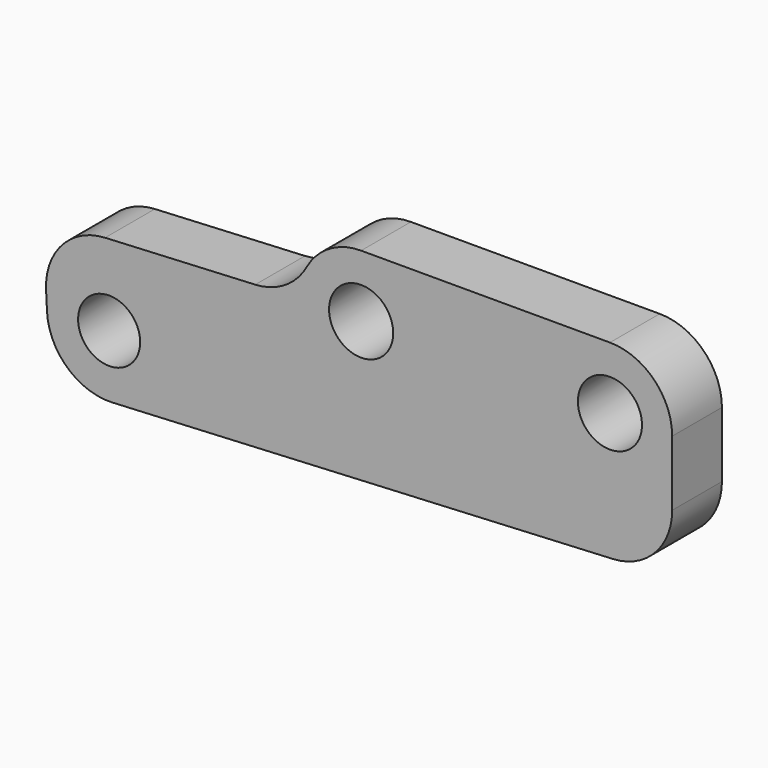
from build123d import *

# Parameters (mm, degrees)
F1_DEPTH = 25.4
F3_D     = 26.1874
F4_R     = 25.4
F7_D     = 25.3492


# Not quite as in the source:
# - a feature names something its author has since deleted; it is built from what else it names


with BuildPart() as f1:
    # F0 (on Front) → F1 (new body)
    with BuildSketch(Plane.XZ):
        Polygon((-177.8, -25.4), (76.2, -12.7), (-76.2, -12.7), (-76.2, 12.7), (-76.2, 38.1), (-180.7137157107, 32.8743142145), align=None)
        Polygon((-76.2, -12.7), (76.2, -12.7), (76.2, 12.7), (50.8, 12.7), (-50.7999999312, 12.7), (-76.2, 12.7), align=None)
        with BuildLine():
            Line((50.8, 12.7), (76.2, 12.7))
            Line((76.2, 12.7), (76.2, 38.1))
            ThreePointArc((76.2, 38.1), (68.7605122421, 20.1394877579), (50.8, 12.7))
        make_face()
        with BuildLine():
            Line((-76.2, 38.1), (-76.2, 12.7))
            Line((-76.2, 12.7), (-50.7999999312, 12.7))
            ThreePointArc((-50.7999999312, 12.7), (-68.7605122178, 20.1394877335), (-76.2, 38.1))
        make_face()
        with BuildLine():
            Line((-50.7999999312, 12.7), (50.8, 12.7))
            ThreePointArc((50.8, 12.7), (25.4, 38.1), (50.8, 63.5))
            Line((50.8, 63.5), (-50.8, 63.5))
            ThreePointArc((-50.8, 63.5), (-32.8394877579, 56.0605122421), (-25.4, 38.1))
            ThreePointArc((-25.4, 38.1), (-32.8394877335, 20.1394877822), (-50.7999999312, 12.7))
        make_face()
        with BuildLine():
            ThreePointArc((50.8, 63.5), (25.4, 38.1), (50.8, 12.7))
            ThreePointArc((50.8, 12.7), (68.7605122421, 20.1394877579), (76.2, 38.1))
            ThreePointArc((76.2, 38.1), (68.7605122421, 56.0605122421), (50.8, 63.5))
        make_face()
        with BuildLine():
            ThreePointArc((-76.2, 38.1), (-68.7605122178, 20.1394877335), (-50.7999999312, 12.7))
            ThreePointArc((-50.7999999312, 12.7), (-32.8394877335, 20.1394877822), (-25.4, 38.1))
            ThreePointArc((-25.4, 38.1), (-32.8394877579, 56.0605122421), (-50.8, 63.5))
            ThreePointArc((-50.8, 63.5), (-68.7605122421, 56.0605122421), (-76.2, 38.1))
        make_face()
    extrude(amount=F1_DEPTH)

    # F3 (through all)
    with Locations(Plane.XZ.offset(25.4)):
        with Locations((-50.8, 38.1), (50.8, 38.1)):
            Hole(F3_D / 2)

    # F4
    f4_edges = [f1.edges().sort_by_distance(p)[0] for p in [
        (76.2, -12.7, -12.7),
        (-177.8, -12.7, -25.4),
        (-76.2, -12.7, 38.1),
        (-180.713716, -12.7, 32.874314),
    ]]
    fillet(f4_edges, radius=F4_R)

    # F7 (through all)
    with Locations(Plane.XZ.offset(25.4)):
        with Locations((-153.7001060629, 1.2367248779)):
            Hole(F7_D / 2)


solid = f1.part
